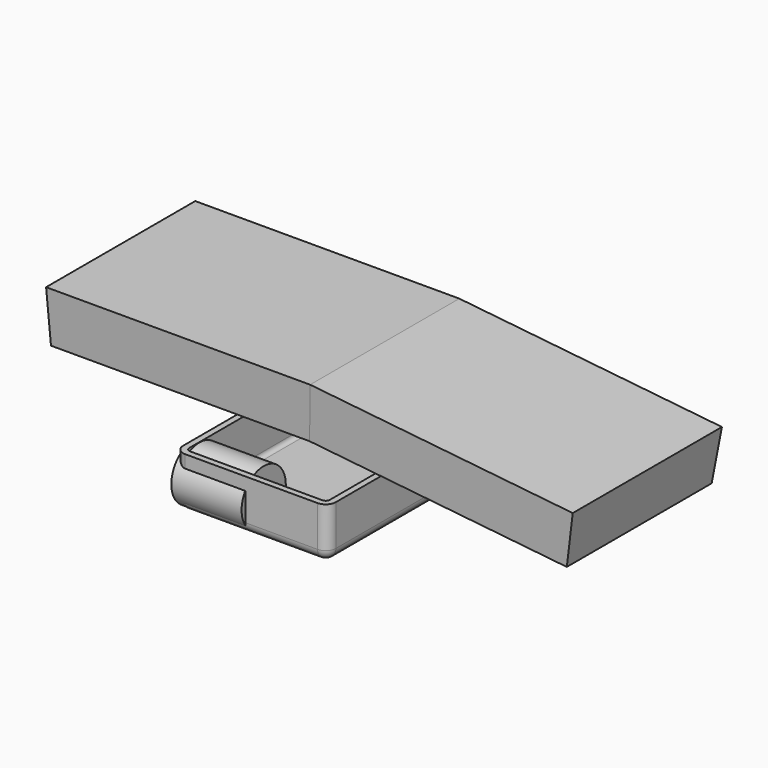
from build123d import *

# Parameters (mm, degrees)
F0_W                   = 254
F0_H                   = 177.8
F1_DEPTH               = 50.8
DRAFT_F1_DRAFTED_ANGLE = -3
F3_R                   = 27.1549962407
F4_DEPTH               = 69
F5_R                   = 12
F6_DEPTH               = 198.6633151876
F13_W                  = 200
F13_H                  = 50
F8_DEPTH               = 150
F9_R                   = 10
F10_T                  = -6


# Not quite as in the source:
# - an extrude with a draft is written as a straight extrude whose walls are then drafted
# - the program builds the solid bodies; features that only make, move or delete a surface that nothing else refers to are left out


with BuildPart() as f1:
    # F0 (on Top) → F1 (new body)
    with BuildSketch(Plane.XY):
        Rectangle(F0_W, F0_H)
    extrude(amount=F1_DEPTH)

    # draft_F1_drafted
    draft_f1_drafted_walls = [f1.faces().sort_by_distance(p)[0] for p in [
        (127, 0, 33.8666666667),
        (0, 88.9, 33.8666666667),
        (-127, 0, 33.8666666667),
        (0, -88.9, 33.8666666667),
    ]]
    draft(draft_f1_drafted_walls, neutral_plane=Plane.XY, angle=DRAFT_F1_DRAFTED_ANGLE)

    # F2: F1 across face


with BuildPart() as f1_1:
    add(f1.part)
    add(f1.part.mirror(Plane(origin=(128.3377036716, 0, 25.5249066057), x_dir=(0, 1, 0), z_dir=(0.9986295348, 0, -0.0523359562))))


with BuildPart() as f4:
    # F3 (on Right) → F4 (new body)
    with BuildSketch(Plane.YZ):
        with Locations((-72.7512463927, -74.0810260177)):
            Circle(F3_R)
    extrude(amount=F4_DEPTH)

    # F5 (on face) → F6 (cut, through all)
    with BuildSketch(Plane.YZ.offset(69)):
        with Locations((-72.7512463927, -74.0810260177)):
            Circle(F5_R)
    extrude(amount=-F6_DEPTH, mode=Mode.SUBTRACT)


with BuildPart() as f8:
    # F13 (on Right) → F8 (new body)
    with BuildSketch(Plane.YZ):
        with Locations((4.6121552587, -71.6192535506)):
            Rectangle(F13_W, F13_H)
    extrude(amount=F8_DEPTH)

    # F9
    f9_edges = [f8.edges().sort_by_distance(p)[0] for p in [
        (0, -95.387845, -71.619254),
        (150, -95.387845, -71.619254),
        (0, 104.612155, -71.619254),
        (150, 104.612155, -71.619254),
        (75, -95.387845, -96.619254),
        (75, 104.612155, -96.619254),
        (0, 4.612155, -96.619254),
        (150, 4.612155, -96.619254),
    ]]
    fillet(f9_edges, radius=F9_R)

    # F10
    f10_openings = [f8.faces().sort_by_distance(p)[0] for p in [
        (75, 4.612155, -46.619254),
    ]]
    offset(amount=F10_T, openings=f10_openings)


solid = Compound([f1_1.part, f4.part, f8.part])
